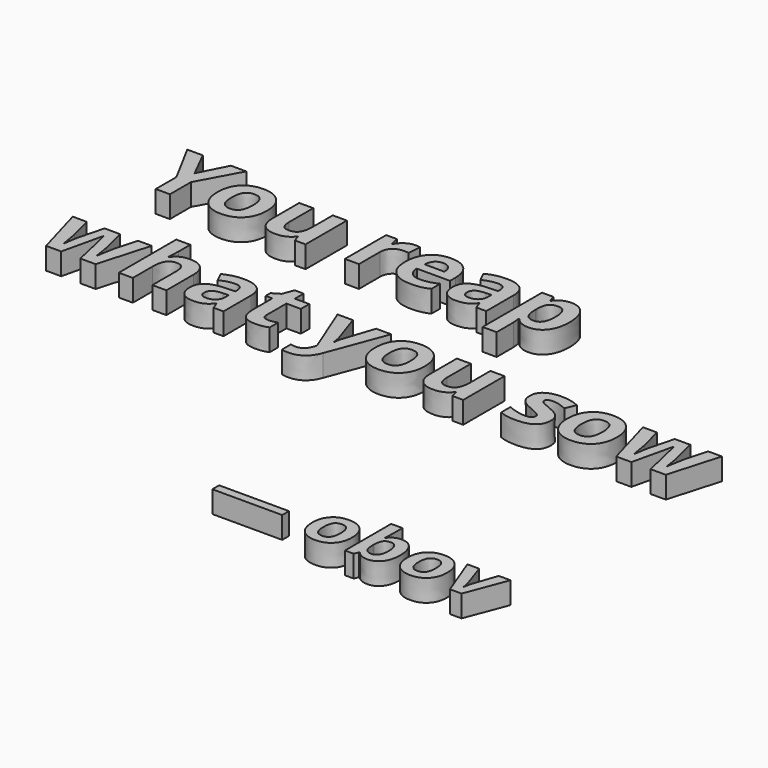
from build123d import *

# Parameters (mm, degrees)
F0_TEXT_SIZE   = 17.2821170593
F0_TEXT_SIZE_2 = 13.8888888889
F1_DEPTH       = 4


# Not quite as in the source:
# - Text() gives the source's letters only with a copy of the font that has no kerning and outlines rounded to 1/6400 em; it was checked with that copy


with BuildPart() as f1:
    # F0 (on Top) → F1 (new body)
    with BuildSketch(Plane.XY):
        with Locations((-59.8431693973, 22.5104912564)):
            Text('You reap', F0_TEXT_SIZE, font='Open Sans', font_style=FontStyle.BOLD, text_align=(TextAlign.LEFT, TextAlign.BOTTOM))
        with Locations((-59.8431693973, -0.9931879443)):
            Text('what you sow', F0_TEXT_SIZE, font='Open Sans', font_style=FontStyle.BOLD, text_align=(TextAlign.LEFT, TextAlign.BOTTOM))
        with Locations((7.9980045557, -47.8889404237)):
            Text('— obov', F0_TEXT_SIZE_2, font='Open Sans', font_style=FontStyle.BOLD, text_align=(TextAlign.LEFT, TextAlign.BOTTOM))
    extrude(amount=F1_DEPTH)


solid = f1.part
